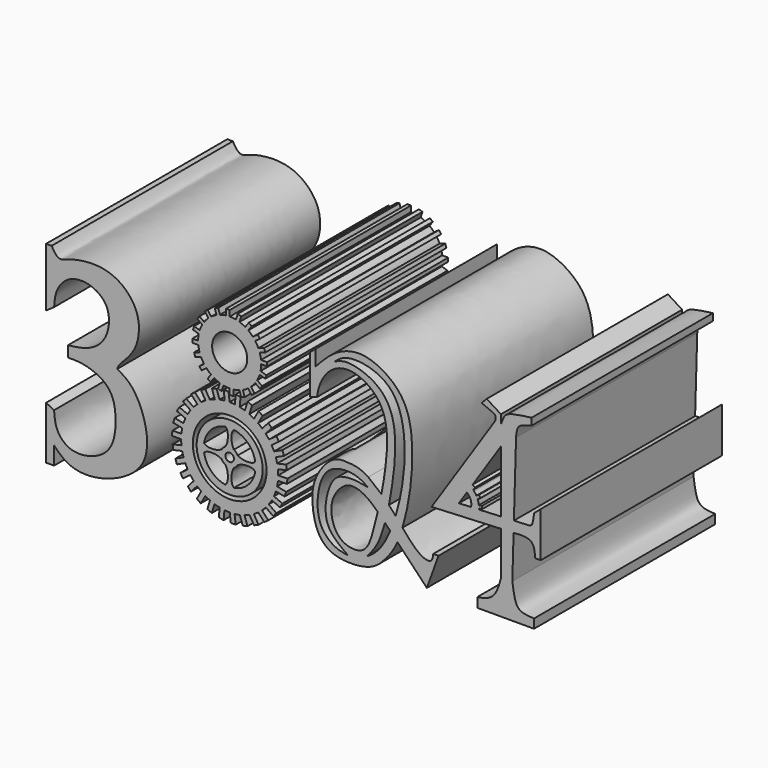
from build123d import *

# Parameters (mm, degrees)
F1_DEPTH = 25.4
F0_R     = 1.9676084545
F0_R_2   = 4.1353313865
F0_R_3   = 3.7014944741
F0_R_4   = 0.4711528495


with BuildPart() as f1:
    # F0 (on Front) → F1 (new body)
    with BuildSketch(Plane.XZ):
        with BuildLine():
            Line((-26.0463822633, -4.2281472124), (-26.9399750978, -3.781349631))
            Line((-26.9399750978, -3.781349631), (-26.9399750978, -9.7014131024))
            Line((-26.9399750978, -9.7014131024), (-26.0463822633, -9.7014131024))
            Line((-26.0463822633, -9.7014131024), (-26.0463822633, -7.6908254996))
            add(Edge.make_bspline(
                [(-26.0463822633, -7.6908254996), (-25.5832112399, -8.1670695829), (-24.5348039921, -9.2450682559), (-21.1768807028, -9.7699938511), (-15.5930362962, -7.2666656298), (-15.4178349045, -2.5163744911), (-17.1134611451, 1.0983060868), (-18.415577289, 1.8388840886), (-18.9613867551, 2.1493129898)],
                knots=[0, 0, 0, 0, 0.129274057, 0.2926173087, 0.50613754, 0.6937062734, 0.8716105194, 1, 1, 1, 1], degree=3))
            add(Edge.make_bspline(
                [(-18.9613867551, 2.1493129898), (-18.9005136877, 2.315911763), (-18.7169213448, 2.8183713956), (-16.6025126501, 4.5351279748), (-16.1925772333, 8.7200429779), (-19.1822179655, 11.5499333245), (-22.3387316619, 11.7305561988), (-24.41055806, 11.26250848), (-25.559395717, 10.6703060682), (-26.056975445, 11.4817221186), (-26.3196341693, 11.9100464508)],
                knots=[0, 0, 0, 0, 0.0677831185, 0.2044329627, 0.3733647654, 0.5392909189, 0.6902206867, 0.8157546293, 0.9027419099, 1, 1, 1, 1], degree=3))
            Line((-26.3196341693, 11.9100464508), (-26.9399750978, 11.9100464508))
            Line((-26.9399750978, 11.9100464508), (-26.9399750978, 5.3211003542))
            Line((-26.9399750978, 5.3211003542), (-26.0422043502, 5.9453165159))
            add(Edge.make_bspline(
                [(-26.0422043502, 5.9453165159), (-26.0009159793, 6.5093417381), (-25.9150413445, 7.6824434828), (-24.6120501776, 9.4535448655), (-22.1715623233, 9.7630392129), (-19.6107393646, 8.1518881576), (-19.9551089552, 4.5626923484), (-22.1437336262, 2.9722513752), (-23.7131036319, 2.7876993587), (-24.4825910777, 2.6972105261)],
                knots=[0, 0, 0, 0, 0.1221770543, 0.2541129544, 0.3944346974, 0.5457596611, 0.710117129, 0.8578657492, 1, 1, 1, 1], degree=3))
            Line((-24.4825910777, 2.6972105261), (-24.4825910777, 1.468517934))
            add(Edge.make_bspline(
                [(-26.0463822633, -4.2281472124), (-25.9967725583, -4.8661935435), (-25.8925157061, -6.2070743666), (-23.9620153869, -8.1304354588), (-19.5761648799, -6.930142804), (-18.9392916703, -3.0716265738), (-19.513902686, 0.3100528568), (-22.6669036758, 1.5162037435), (-23.9313084782, 1.4829963938), (-24.4825910777, 1.468517934)],
                knots=[0, 0, 0, 0, 0.1192071231, 0.2505187124, 0.418191993, 0.5811975133, 0.7349402199, 0.8844334945, 1, 1, 1, 1], degree=3))
        make_face()
    extrude(amount=F1_DEPTH)


with BuildPart() as f1b:
    # F0 (on Front) → F1, piece 2 (new body)
    with BuildSketch(Plane.XZ):
        with BuildLine():
            Line((-9.1431848754, 11.0277357752), (-8.7476742344, 10.4833620795))
            ThreePointArc((-8.7476742344, 10.4833620795), (-8.9926500243, 10.2350100375), (-9.2119951729, 9.9637544749))
            Line((-9.2119951729, 9.9637544749), (-9.7375776543, 10.3456124996))
            Line((-9.7375776543, 10.3456124996), (-9.9805512287, 10.0111880646))
            Line((-9.9805512287, 10.0111880646), (-9.436177533, 9.6156774235))
            ThreePointArc((-9.436177533, 9.6156774235), (-9.5924183528, 9.3037789133), (-9.717205407, 8.9780181644))
            Line((-9.717205407, 8.9780181644), (-10.3350646698, 9.1787728084))
            Line((-10.3350646698, 9.1787728084), (-10.4628034373, 8.7856333066))
            Line((-10.4628034373, 8.7856333066), (-9.8228537772, 8.5777010574))
            ThreePointArc((-9.8228537772, 8.5777010574), (-9.8750656868, 8.2327868784), (-9.8930796203, 7.8844086749))
            Line((-9.8930796203, 7.8844086749), (-10.5427352951, 7.8844086749))
            Line((-10.5427352951, 7.8844086749), (-10.5427352951, 7.4710373399))
            Line((-10.5427352951, 7.4710373399), (-9.8698524021, 7.4710373399))
            ThreePointArc((-9.8698524021, 7.4710373399), (-9.812924536, 7.126870095), (-9.7224020195, 6.7899761229))
            Line((-9.7224020195, 6.7899761229), (-10.3402612823, 6.5892214788))
            Line((-10.3402612823, 6.5892214788), (-10.2125225148, 6.196081977))
            Line((-10.2125225148, 6.196081977), (-9.5725728547, 6.4040142262))
            ThreePointArc((-9.5725728547, 6.4040142262), (-9.4120777091, 6.0942834033), (-9.2218797172, 5.8018511918))
            Line((-9.2218797172, 5.8018511918), (-9.7474621987, 5.4199931671))
            Line((-9.7474621987, 5.4199931671), (-9.5044886242, 5.0855687321))
            Line((-9.5044886242, 5.0855687321), (-8.9601149285, 5.4810793731))
            ThreePointArc((-8.9601149285, 5.4810793731), (-8.7117628865, 5.2361035832), (-8.4405073239, 5.0167584346))
            Line((-8.4405073239, 5.0167584346), (-8.8223653486, 4.4911759532))
            Line((-8.8223653486, 4.4911759532), (-8.4879409136, 4.2482023788))
            Line((-8.4879409136, 4.2482023788), (-8.0924302726, 4.7925760745))
            ThreePointArc((-8.0924302726, 4.7925760745), (-7.7805317624, 4.6363352547), (-7.4547710134, 4.5115482005))
            Line((-7.4547710134, 4.5115482005), (-7.6555256574, 3.8936889377))
            Line((-7.6555256574, 3.8936889377), (-7.2623861556, 3.7659501702))
            Line((-7.2623861556, 3.7659501702), (-7.0544539065, 4.4058998303))
            ThreePointArc((-7.0544539065, 4.4058998303), (-6.7095397274, 4.3536879207), (-6.3611615239, 4.3356739872))
            Line((-6.3611615239, 4.3356739872), (-6.3611615239, 3.6860183124))
            Line((-6.3611615239, 3.6860183124), (-5.9477901889, 3.6860183124))
            Line((-5.9477901889, 3.6860183124), (-5.9477901889, 4.3589012054))
            ThreePointArc((-5.9477901889, 4.3589012054), (-5.603622944, 4.4158290715), (-5.2667289719, 4.506351588))
            Line((-5.2667289719, 4.506351588), (-5.0659743279, 3.8884923252))
            Line((-5.0659743279, 3.8884923252), (-4.6728348261, 4.0162310927))
            Line((-4.6728348261, 4.0162310927), (-4.8807670752, 4.6561807528))
            ThreePointArc((-4.8807670752, 4.6561807528), (-4.5710362523, 4.8166758984), (-4.2786040408, 5.0068738902))
            Line((-4.2786040408, 5.0068738902), (-3.8967460161, 4.4812914088))
            Line((-3.8967460161, 4.4812914088), (-3.5623215811, 4.7242649833))
            Line((-3.5623215811, 4.7242649833), (-3.9578322221, 5.268638679))
            ThreePointArc((-3.9578322221, 5.268638679), (-3.7128564322, 5.516990721), (-3.4935112837, 5.7882462836))
            Line((-3.4935112837, 5.7882462836), (-2.9679288023, 5.4063882589))
            Line((-2.9679288023, 5.4063882589), (-2.7249552278, 5.7408126939))
            Line((-2.7249552278, 5.7408126939), (-3.2693289235, 6.1363233349))
            ThreePointArc((-3.2693289235, 6.1363233349), (-3.1130881037, 6.4482218451), (-2.9883010496, 6.7739825941))
            Line((-2.9883010496, 6.7739825941), (-2.3704417867, 6.5732279501))
            Line((-2.3704417867, 6.5732279501), (-2.2427030192, 6.9663674519))
            Line((-2.2427030192, 6.9663674519), (-2.8826526793, 7.174299701))
            ThreePointArc((-2.8826526793, 7.174299701), (-2.8304407697, 7.5192138801), (-2.8124268362, 7.8675920836))
            Line((-2.8124268362, 7.8675920836), (-2.1627711614, 7.8675920836))
            Line((-2.1627711614, 7.8675920836), (-2.1627711614, 8.2809634186))
            Line((-2.1627711614, 8.2809634186), (-2.8356540545, 8.2809634186))
            ThreePointArc((-2.8356540545, 8.2809634186), (-2.8925819205, 8.6251306635), (-2.983104437, 8.9620246356))
            Line((-2.983104437, 8.9620246356), (-2.3652451742, 9.1627792796))
            Line((-2.3652451742, 9.1627792796), (-2.4929839417, 9.5559187814))
            Line((-2.4929839417, 9.5559187814), (-3.1329336018, 9.3479865323))
            ThreePointArc((-3.1329336018, 9.3479865323), (-3.2934287474, 9.6577173552), (-3.4836267393, 9.9501495667))
            Line((-3.4836267393, 9.9501495667), (-2.9580442579, 10.3320075914))
            Line((-2.9580442579, 10.3320075914), (-3.2010178323, 10.6664320264))
            Line((-3.2010178323, 10.6664320264), (-3.745391528, 10.2709213854))
            ThreePointArc((-3.745391528, 10.2709213854), (-3.99374357, 10.5158971753), (-4.2649991326, 10.7352423238))
            Line((-4.2649991326, 10.7352423238), (-3.8831411079, 11.2608248052))
            Line((-3.8831411079, 11.2608248052), (-4.2175655429, 11.5037983797))
            Line((-4.2175655429, 11.5037983797), (-4.613076184, 10.959424684))
            ThreePointArc((-4.613076184, 10.959424684), (-4.9249746942, 11.1156655038), (-5.2507354431, 11.2404525579))
            Line((-5.2507354431, 11.2404525579), (-5.0499807991, 11.8583118208))
            Line((-5.0499807991, 11.8583118208), (-5.4431203009, 11.9860505883))
            Line((-5.4431203009, 11.9860505883), (-5.6510525501, 11.3461009282))
            ThreePointArc((-5.6510525501, 11.3461009282), (-5.9959667291, 11.3983128378), (-6.3443449326, 11.4163267713))
            Line((-6.3443449326, 11.4163267713), (-6.3443449326, 11.393099553))
            Line((-6.3443449326, 11.393099553), (-6.7577162676, 11.393099553))
            ThreePointArc((-6.7577162676, 11.393099553), (-7.1018835125, 11.336171687), (-7.4387774846, 11.2456491705))
            Line((-7.4387774846, 11.2456491705), (-7.6395321286, 11.8635084333))
            Line((-7.6395321286, 11.8635084333), (-8.0326716305, 11.7357696658))
            Line((-8.0326716305, 11.7357696658), (-7.8247393813, 11.0958200057))
            ThreePointArc((-7.8247393813, 11.0958200057), (-8.1344702042, 10.9353248601), (-8.4269024157, 10.7451268682))
            Line((-8.4269024157, 10.7451268682), (-8.8087604404, 11.2707093496))
            Line((-8.8087604404, 11.2707093496), (-9.1431848754, 11.0277357752))
        make_face()
        with Locations((-6.3527532283, 7.8760003792)):
            Circle(F0_R, mode=Mode.SUBTRACT)
        Polygon((-6.7577162676, 12.0659824461), (-6.7577162676, 11.393099553), (-6.3443449326, 11.393099553), (-6.3443449326, 11.4163267713), (-6.3443449326, 12.0659824461), align=None)
    extrude(amount=F1_DEPTH)


with BuildPart() as f1c:
    # F0 (on Front) → F1, piece 3 (new body)
    with BuildSketch(Plane.XZ):
        with BuildLine():
            Line((-8.3493689741, 3.6920308456), (-8.0175920904, 2.7096574241))
            ThreePointArc((-8.0175920904, 2.7096574241), (-8.2983395388, 2.6108656256), (-8.5732644732, 2.4968690045))
            Line((-8.5732644732, 2.4968690045), (-9.087648101, 3.3645220331))
            Line((-9.087648101, 3.3645220331), (-9.5868565309, 3.1422601201))
            Line((-9.5868565309, 3.1422601201), (-9.0580828491, 2.2503342077))
            ThreePointArc((-9.0580828491, 2.2503342077), (-9.3121553223, 2.0953305703), (-9.5573712571, 1.926664941))
            Line((-9.5573712571, 1.926664941), (-10.2409095766, 2.6684112994))
            Line((-10.2409095766, 2.6684112994), (-10.6829982545, 2.3472150737))
            Line((-10.6829982545, 2.3472150737), (-9.9803377218, 1.5847181127))
            ThreePointArc((-9.9803377218, 1.5847181127), (-10.1966310335, 1.3802770392), (-10.4014208556, 1.1643138989))
            Line((-10.4014208556, 1.1643138989), (-11.2242399624, 1.747735712))
            Line((-11.2242399624, 1.747735712), (-11.5898874916, 1.34164299))
            Line((-11.5898874916, 1.34164299), (-10.744049745, 0.7418997564))
            ThreePointArc((-10.744049745, 0.7418997564), (-10.9131108396, 0.4969563028), (-11.0685242511, 0.243134277))
            Line((-11.0685242511, 0.243134277), (-11.9946630019, 0.642733212))
            Line((-11.9946630019, 0.642733212), (-12.2678888309, 0.1694921942))
            Line((-12.2678888309, 0.1694921942), (-11.3158410386, -0.2412856547))
            ThreePointArc((-11.3158410386, -0.2412856547), (-11.4302811351, -0.5160262842), (-11.5295258242, -0.7966139548))
            Line((-11.5295258242, -0.7966139548), (-12.5185075114, -0.598302289))
            Line((-12.5185075114, -0.598302289), (-12.6873703603, -1.1180086992))
            Line((-12.6873703603, -1.1180086992), (-11.6707215794, -1.3218682002))
            ThreePointArc((-11.6707215794, -1.3218682002), (-11.7255390964, -1.6143985218), (-11.7642775939, -1.9094888097))
            Line((-11.7642775939, -1.9094888097), (-12.7728789721, -1.9211315843))
            Line((-12.7728789721, -1.9211315843), (-12.8299987242, -2.464589723))
            Line((-12.8299987242, -2.464589723), (-11.7931813849, -2.4526212379))
            ThreePointArc((-11.7931813849, -2.4526212379), (-11.7859805338, -2.7501562727), (-11.7625197814, -3.0468523164))
            Line((-11.7625197814, -3.0468523164), (-12.7466601307, -3.2679406863))
            Line((-12.7466601307, -3.2679406863), (-12.6895403787, -3.811398825))
            Line((-12.6895403787, -3.811398825), (-11.6778683738, -3.5841254339))
            ThreePointArc((-11.6778683738, -3.5841254339), (-11.6089638664, -3.8736614732), (-11.5243292117, -4.1589962317))
            Line((-11.5243292117, -4.1589962317), (-12.4409968763, -4.5798675744))
            Line((-12.4409968763, -4.5798675744), (-12.2721340274, -5.0995739846))
            Line((-12.2721340274, -5.0995739846), (-11.3298222781, -4.6669286253))
            ThreePointArc((-11.3298222781, -4.6669286253), (-11.202225572, -4.9358115549), (-11.0601159554, -5.1973145302))
            Line((-11.0601159554, -5.1973145302), (-11.8692481598, -5.7995747482))
            Line((-11.8692481598, -5.7995747482), (-11.5960223308, -6.272815766))
            Line((-11.5960223308, -6.272815766), (-10.7642543823, -5.6537071168))
            ThreePointArc((-10.7642543823, -5.6537071168), (-10.5835420658, -5.8901854623), (-10.3901683596, -6.1164277195))
            Line((-10.3901683596, -6.1164277195), (-11.0564021437, -6.8737551516))
            Line((-11.0564021437, -6.8737551516), (-10.6907546145, -7.2798478736))
            Line((-10.6907546145, -7.2798478736), (-10.0058827173, -6.5013339532))
            ThreePointArc((-10.0058827173, -6.5013339532), (-9.7799527859, -6.6950724763), (-9.5437663489, -6.8761661431))
            Line((-9.5437663489, -6.8761661431), (-10.0379840994, -7.7554619463))
            Line((-10.0379840994, -7.7554619463), (-9.5958954215, -8.076658172))
            Line((-9.5958954215, -8.076658172), (-9.087851764, -7.1727637745))
            ThreePointArc((-9.087851764, -7.1727637745), (-8.8265784398, -7.3152951719), (-8.5579017526, -7.4433255862))
            Line((-8.5579017526, -7.4433255862), (-8.8585037824, -8.4061603146))
            Line((-8.8585037824, -8.4061603146), (-8.3592953524, -8.6284222275))
            Line((-8.3592953524, -8.6284222275), (-8.0502838802, -7.6386518755))
            ThreePointArc((-8.0502838802, -7.6386518755), (-7.7650860612, -7.7237468413), (-7.4756615843, -7.7931184595))
            Line((-7.4756615843, -7.7931184595), (-7.5695101422, -8.7974116153))
            Line((-7.5695101422, -8.7974116153), (-7.034999764, -8.9110253034))
            Line((-7.034999764, -8.9110253034), (-6.9385257613, -7.8786367106))
            ThreePointArc((-6.9385257613, -7.8786367106), (-6.6418679606, -7.9025761865), (-6.3443449326, -7.9102571361))
            Line((-6.3443449326, -7.9102571361), (-6.2273383862, -8.9121162891))
            Line((-6.2273383862, -8.9121162891), (-5.6808867282, -8.9121162891))
            Line((-5.6808867282, -8.9121162891), (-5.8011665719, -7.882229791))
            ThreePointArc((-5.8011665719, -7.882229791), (-5.506014159, -7.843967507), (-5.2133957637, -7.7896220936))
            Line((-5.2133957637, -7.7896220936), (-4.8906478606, -8.7452611915))
            Line((-4.8906478606, -8.7452611915), (-4.3561374824, -8.6316475034))
            Line((-4.3561374824, -8.6316475034), (-4.6879143661, -7.6492740819))
            ThreePointArc((-4.6879143661, -7.6492740819), (-4.4071669178, -7.5504822834), (-4.1322419833, -7.4364856623))
            Line((-4.1322419833, -7.4364856623), (-3.6178583556, -8.3041386909))
            Line((-3.6178583556, -8.3041386909), (-3.1186499256, -8.0818767779))
            Line((-3.1186499256, -8.0818767779), (-3.6474236074, -7.1899508655))
            ThreePointArc((-3.6474236074, -7.1899508655), (-3.3933511342, -7.0349472281), (-3.1481351994, -6.8662815988))
            Line((-3.1481351994, -6.8662815988), (-2.4645968799, -7.6080279572))
            Line((-2.4645968799, -7.6080279572), (-2.022508202, -7.2868317315))
            Line((-2.022508202, -7.2868317315), (-2.7251687347, -6.5243347705))
            ThreePointArc((-2.7251687347, -6.5243347705), (-2.508875423, -6.319893697), (-2.3040856009, -6.1039305567))
            Line((-2.3040856009, -6.1039305567), (-1.4812664942, -6.6873523698))
            Line((-1.4812664942, -6.6873523698), (-1.1156189649, -6.2812596477))
            Line((-1.1156189649, -6.2812596477), (-1.9614567115, -5.6815164142))
            ThreePointArc((-1.9614567115, -5.6815164142), (-1.7923956169, -5.4365729606), (-1.6369822054, -5.1827509348))
            Line((-1.6369822054, -5.1827509348), (-0.7108434547, -5.5823498698))
            Line((-0.7108434547, -5.5823498698), (-0.4376176257, -5.109108852))
            Line((-0.4376176257, -5.109108852), (-1.3896654179, -4.6983310031))
            ThreePointArc((-1.3896654179, -4.6983310031), (-1.2752253214, -4.4235903736), (-1.1759806323, -4.143002703))
            Line((-1.1759806323, -4.143002703), (-0.1869989452, -4.3413143688))
            Line((-0.1869989452, -4.3413143688), (-0.0181360962, -3.8216079586))
            Line((-0.0181360962, -3.8216079586), (-1.0347848771, -3.6177484575))
            ThreePointArc((-1.0347848771, -3.6177484575), (-0.9799673601, -3.325218136), (-0.9412288626, -3.030127848))
            Line((-0.9412288626, -3.030127848), (0.0673725156, -3.0184850734))
            Line((0.0673725156, -3.0184850734), (0.1244922677, -2.4750269348))
            Line((0.1244922677, -2.4750269348), (-0.9123250717, -2.4869954199))
            ThreePointArc((-0.9123250717, -2.4869954199), (-0.9195259227, -2.1894603851), (-0.9429866751, -1.8927643414))
            Line((-0.9429866751, -1.8927643414), (0.0411536742, -1.6716759715))
            Line((0.0411536742, -1.6716759715), (-0.0159660779, -1.1282178328))
            Line((-0.0159660779, -1.1282178328), (-1.0276380828, -1.3554912239))
            ThreePointArc((-1.0276380828, -1.3554912239), (-1.0965425901, -1.0659551846), (-1.1811772449, -0.7806204261))
            Line((-1.1811772449, -0.7806204261), (-0.2645095802, -0.3597490834))
            Line((-0.2645095802, -0.3597490834), (-0.4333724292, 0.1599573268))
            Line((-0.4333724292, 0.1599573268), (-1.3756841785, -0.2726880325))
            ThreePointArc((-1.3756841785, -0.2726880325), (-1.5032808845, -0.0038051029), (-1.6453905011, 0.2576978724))
            Line((-1.6453905011, 0.2576978724), (-0.8362582967, 0.8599580905))
            Line((-0.8362582967, 0.8599580905), (-1.1094841257, 1.3331991082))
            Line((-1.1094841257, 1.3331991082), (-1.9412520743, 0.714090459))
            ThreePointArc((-1.9412520743, 0.714090459), (-2.1219643907, 0.9505688045), (-2.3153380969, 1.1768110617))
            Line((-2.3153380969, 1.1768110617), (-1.6491043128, 1.9341384938))
            Line((-1.6491043128, 1.9341384938), (-2.0147518421, 2.3402312158))
            Line((-2.0147518421, 2.3402312158), (-2.6996237392, 1.5617172954))
            ThreePointArc((-2.6996237392, 1.5617172954), (-2.9255536706, 1.7554558185), (-3.1617401076, 1.9365494853))
            Line((-3.1617401076, 1.9365494853), (-2.6675223571, 2.8158452885))
            Line((-2.6675223571, 2.8158452885), (-3.109611035, 3.1370415142))
            Line((-3.109611035, 3.1370415142), (-3.6176546925, 2.2331471167))
            ThreePointArc((-3.6176546925, 2.2331471167), (-3.8789280167, 2.3756785141), (-4.1476047039, 2.5037089284))
            Line((-4.1476047039, 2.5037089284), (-3.8470026741, 3.4665436568))
            Line((-3.8470026741, 3.4665436568), (-4.3462111041, 3.6888055697))
            Line((-4.3462111041, 3.6888055697), (-4.6552225763, 2.6990352177))
            ThreePointArc((-4.6552225763, 2.6990352177), (-4.9404203953, 2.7841301835), (-5.2298448722, 2.8535018017))
            Line((-5.2298448722, 2.8535018017), (-5.1359963143, 3.8577949575))
            Line((-5.1359963143, 3.8577949575), (-5.6705066925, 3.9714086456))
            Line((-5.6705066925, 3.9714086456), (-5.7669806952, 2.9390200528))
            ThreePointArc((-5.7669806952, 2.9390200528), (-6.0636384959, 2.9629595287), (-6.3611615239, 2.9706404783))
            Line((-6.3611615239, 2.9706404783), (-6.4781680703, 3.9724996313))
            Line((-6.4781680703, 3.9724996313), (-7.0246197283, 3.9724996313))
            Line((-7.0246197283, 3.9724996313), (-6.9043398847, 2.9426131332))
            ThreePointArc((-6.9043398847, 2.9426131332), (-7.1994922975, 2.9043508492), (-7.4921106928, 2.8500054358))
            Line((-7.4921106928, 2.8500054358), (-7.8148585959, 3.8056445337))
            Line((-7.8148585959, 3.8056445337), (-8.3493689741, 3.6920308456))
        make_face()
        with Locations((-6.3527532283, -2.4698083289)):
            Circle(F0_R_2, mode=Mode.SUBTRACT)
    extrude(amount=F1_DEPTH)


with BuildPart() as f1d:
    # F0 (on Front) → F1, piece 4 (new body)
    with BuildSketch(Plane.XZ):
        with Locations((-6.3527532283, -2.4698083289)):
            Circle(F0_R_3)
        with BuildLine():
            add(Edge.make_bspline(
                [(-7.2560629998, -2.9409611784), (-7.4238569383, -2.8554461757), (-7.8043314459, -2.6615400144), (-8.8419767294, -2.6416756573), (-9.1140801532, -2.8547030748), (-9.2242590475, -2.9409611784)],
                knots=[0, 0, 0, 0, 0.3194921696, 0.7244518306, 1, 1, 1, 1], degree=3))
            ThreePointArc((-7.2560629998, -2.9409611784), (-7.0731536554, -3.1902087561), (-6.8239060777, -3.3731181005))
            add(Edge.make_bspline(
                [(-6.8239060777, -3.3731181005), (-6.7383910751, -3.5409120389), (-6.5444849137, -3.9213865465), (-6.5246205566, -4.9590318301), (-6.7376479741, -5.2311352538), (-6.8239060777, -5.3413141481)],
                knots=[0, 0, 0, 0, 0.3194921696, 0.7244518306, 1, 1, 1, 1], degree=3))
            ThreePointArc((-6.8239060777, -5.3413141481), (-8.4103647899, -4.5274198906), (-9.2242590475, -2.9409611784))
        make_face(mode=Mode.SUBTRACT)
        with Locations((-6.3527532283, -2.4698083289)):
            Circle(F0_R_4, mode=Mode.SUBTRACT)
        with BuildLine():
            add(Edge.make_bspline(
                [(-5.8816003788, -3.3731181005), (-5.9671153814, -3.5409120389), (-6.1610215428, -3.9213865465), (-6.1808858999, -4.9590318301), (-5.9678584824, -5.2311352538), (-5.8816003788, -5.3413141481)],
                knots=[0, 0, 0, 0, 0.3194921696, 0.7244518306, 1, 1, 1, 1], degree=3))
            ThreePointArc((-5.8816003788, -3.3731181005), (-5.6323528011, -3.1902087561), (-5.4494434567, -2.9409611784))
            add(Edge.make_bspline(
                [(-5.4494434567, -2.9409611784), (-5.2816495182, -2.8554461757), (-4.9011750106, -2.6615400144), (-3.8635297271, -2.6416756573), (-3.5914263033, -2.8547030748), (-3.481247409, -2.9409611784)],
                knots=[0, 0, 0, 0, 0.3194921696, 0.7244518306, 1, 1, 1, 1], degree=3))
            ThreePointArc((-3.481247409, -2.9409611784), (-4.2951416666, -4.5274198906), (-5.8816003788, -5.3413141481))
        make_face(mode=Mode.SUBTRACT)
        with BuildLine():
            ThreePointArc((-9.2242590475, -1.9986554794), (-8.4103647899, -0.4121967672), (-6.8239060777, 0.4016974903))
            add(Edge.make_bspline(
                [(-6.8239060777, -1.5664985573), (-6.7383910751, -1.3987046188), (-6.5444849137, -1.0182301113), (-6.5246205566, 0.0194151723), (-6.7376479741, 0.2915185961), (-6.8239060777, 0.4016974903)],
                knots=[0, 0, 0, 0, 0.3194921696, 0.7244518306, 1, 1, 1, 1], degree=3))
            ThreePointArc((-6.8239060777, -1.5664985573), (-7.0731536554, -1.7494079017), (-7.2560629998, -1.9986554794))
            add(Edge.make_bspline(
                [(-7.2560629998, -1.9986554794), (-7.4238569383, -2.0841704821), (-7.8043314459, -2.2780766434), (-8.8419767294, -2.2979410005), (-9.1140801532, -2.084913583), (-9.2242590475, -1.9986554794)],
                knots=[0, 0, 0, 0, 0.3194921696, 0.7244518306, 1, 1, 1, 1], degree=3))
        make_face(mode=Mode.SUBTRACT)
        with BuildLine():
            ThreePointArc((-5.4494434567, -1.9986554794), (-5.6323528011, -1.7494079017), (-5.8816003788, -1.5664985573))
            add(Edge.make_bspline(
                [(-5.8816003788, -1.5664985573), (-5.9671153814, -1.3987046188), (-6.1610215428, -1.0182301113), (-6.1808858999, 0.0194151723), (-5.9678584824, 0.2915185961), (-5.8816003788, 0.4016974903)],
                knots=[0, 0, 0, 0, 0.3194921696, 0.7244518306, 1, 1, 1, 1], degree=3))
            ThreePointArc((-5.8816003788, 0.4016974903), (-4.2951416666, -0.4121967672), (-3.481247409, -1.9986554794))
            add(Edge.make_bspline(
                [(-5.4494434567, -1.9986554794), (-5.2816495182, -2.0841704821), (-4.9011750106, -2.2780766434), (-3.8635297271, -2.2979410005), (-3.5914263033, -2.084913583), (-3.481247409, -1.9986554794)],
                knots=[0, 0, 0, 0, 0.3194921696, 0.7244518306, 1, 1, 1, 1], degree=3))
        make_face(mode=Mode.SUBTRACT)
    extrude(amount=F1_DEPTH)


with BuildPart() as f1e:
    # F0 (on Front) → F1, piece 5 (new body)
    with BuildSketch(Plane.XZ):
        with BuildLine():
            Line((2.6719989255, 10.845345445), (2.6719989255, 6.3930512406))
            Line((2.6719989255, 6.3930512406), (3.435845949, 6.6561674627))
            add(Edge.make_bspline(
                [(3.435845949, 6.6561674627), (3.4947846069, 7.0290440395), (3.631181329, 7.891960582), (4.6469745705, 9.8721275201), (7.2502428175, 10.9905601524), (11.4292677124, 8.5643622597), (11.4047338514, 3.7879569996), (10.8541188192, 0.4220713966), (10.662418889, -0.5672860666)],
                knots=[0, 0, 0, 0, 0.0554862745, 0.1284071651, 0.2079981655, 0.3080730139, 0.4305049606, 0.4841391387, 0.4841391387, 0.4841391387, 0.4841391387], degree=3))
            add(Edge.make_bspline(
                [(11.5063009471, -1.3741382079), (11.2197324238, -1.0774084626), (10.9391479112, -0.8121944395), (10.6624189097, -0.5672860636)],
                knots=[0.7225338292, 0.7225338292, 0.7225338292, 0.7225338292, 0.8212279518, 0.8212279518, 0.8212279518, 0.8212279518], degree=3))
            add(Edge.make_bspline(
                [(5.3971023299, 10.8085060492), (5.7772404462, 10.972500295), (6.6584668398, 11.3526675333), (8.9599957978, 10.8384738524), (11.1535014908, 9.4534977213), (12.5082732699, 6.2739507893), (12.0837887958, 1.7807829115), (11.5957909908, -0.9246608458), (11.5063009471, -1.3741382079)],
                knots=[0, 0, 0, 0, 0.0918839164, 0.2130029292, 0.3401946496, 0.4838683251, 0.688082351, 0.7299642077, 0.7299642077, 0.7299642077, 0.7299642077], degree=3))
            add(Edge.make_bspline(
                [(5.3971023299, 10.8085060492), (5.7620619847, 11.1079679478), (6.609363119, 11.8051385726), (9.3198931691, 11.7283905399), (12.668565724, 10.0341568395), (13.6683514535, 4.5184758873), (12.8192457315, -0.3650505129), (12.261372983, -2.2119843023)],
                knots=[0, 0, 0, 0, 0.1014740063, 0.2350549924, 0.3880747556, 0.5958223129, 0.7618945915, 0.7618945915, 0.7618945915, 0.7618945915], degree=3))
            add(Edge.make_bspline(
                [(13.0264212728, -3.1206628495), (12.7704039085, -2.8165986405), (12.5144389833, -2.5076877064), (12.261372983, -2.2119843023)],
                knots=[0.5530933365, 0.5530933365, 0.5530933365, 0.5530933365, 0.6373963086, 0.6373963086, 0.6373963086, 0.6373963086], degree=3))
            add(Edge.make_bspline(
                [(13.0264212728, -3.1206628495), (13.0837947511, -2.9258450596), (13.4575273646, -1.5863706141), (14.0352558584, 1.2503294705), (14.2882363414, 6.1221826163), (13.2278084517, 10.4171777534), (8.9691725141, 12.9168064821), (6.1016622002, 12.1680848808), (4.5226306163, 10.9638438122), (3.6928214025, 10.0698512074), (3.2855544844, 9.6310833469)],
                knots=[0.5451714575, 0.5451714575, 0.5451714575, 0.5451714575, 0.5569891983, 0.6250982674, 0.7020008511, 0.773863392, 0.847306886, 0.9050067166, 0.9533388622, 1, 1, 1, 1], degree=3))
            Line((3.2855544844, 9.6310833469), (3.2855544844, 11.3618402075))
            Line((3.2855544844, 11.3618402075), (2.6719989255, 10.845345445))
        make_face()
        with BuildLine():
            add(Edge.make_bspline(
                [(10.662418889, -0.5672860666), (10.5354882317, -1.2223712975), (10.3980492387, -1.8616839287), (10.2575550909, -2.466147512)],
                knots=[0.4841391387, 0.4841391387, 0.4841391387, 0.4841391387, 0.519652044, 0.519652044, 0.519652044, 0.519652044], degree=3))
            add(Edge.make_bspline(
                [(10.6624189097, -0.5672860636), (10.1611589652, -0.1236651991), (9.6725492558, 0.253331238), (9.1839395463, 0.630327675)],
                knots=[0.8212279518, 0.8212279518, 0.8212279518, 0.8212279518, 1, 1, 1, 1], degree=3))
            add(Edge.make_bspline(
                [(9.1839395463, 0.630327675), (8.3293113858, 1.2043820461), (7.0371029965, 1.3526036912), (5.0848852762, 1.4045628888), (2.9521080111, -1.3902184626), (2.8538912632, -4.0498435296), (3.2760692481, -6.416794074), (4.8429420361, -8.6433503566), (9.3575740444, -8.6163306128), (11.0399209282, -6.984464507), (11.9734456221, -5.7662631109), (12.3803034392, -4.9061127741), (12.4598010347, -4.7229557439)],
                knots=[0, 0, 0, 0, 0.0530742276, 0.0986896089, 0.1608436336, 0.217710048, 0.2707461549, 0.3252123246, 0.3955657221, 0.4477864087, 0.4977663247, 0.5106388975, 0.5106388975, 0.5106388975, 0.5106388975], degree=3))
            add(Edge.make_bspline(
                [(12.4598010347, -4.7229557439), (12.1935596674, -4.4485073887), (11.9253475631, -4.171569745), (11.6621594556, -3.8986119129)],
                knots=[0.448384843, 0.448384843, 0.448384843, 0.448384843, 0.5312386615, 0.5312386615, 0.5312386615, 0.5312386615], degree=3))
            add(Edge.make_bspline(
                [(11.6621594556, -3.8986119129), (11.5577343223, -4.1480369004), (10.7999785534, -5.8142653195), (9.895978436, -6.779659418), (9.0104155242, -7.2580603883)],
                knots=[0.8160688803, 0.8160688803, 0.8160688803, 0.8160688803, 0.8422565533, 1, 1, 1, 1], degree=3))
            add(Edge.make_bspline(
                [(11.0650681475, -3.2797242735), (10.837325615, -4.1199552873), (10.2295225901, -5.8875703382), (9.4570090084, -6.7560110248), (9.0104155242, -7.2580603883)],
                knots=[0.7921233606, 0.7921233606, 0.7921233606, 0.7921233606, 0.8798256046, 1, 1, 1, 1], degree=3))
            add(Edge.make_bspline(
                [(11.0650681475, -3.2797242735), (10.7861687813, -2.99207196), (10.515826503, -2.7171147888), (10.2575550909, -2.466147512)],
                knots=[0.594962196, 0.594962196, 0.594962196, 0.594962196, 0.6859914774, 0.6859914774, 0.6859914774, 0.6859914774], degree=3))
        make_face()
        with BuildLine():
            add(Edge.make_bspline(
                [(10.2575550909, -2.466147512), (9.8682447349, -2.087847184), (9.0400940624, -1.3468679748), (8.4186032489, -1.093940724), (8.0686900765, -0.9515370475)],
                knots=[0.6859914774, 0.6859914774, 0.6859914774, 0.6859914774, 0.8232062069, 1, 1, 1, 1], degree=3))
            add(Edge.make_bspline(
                [(10.2575550909, -2.466147512), (10.0773075767, -3.2416464209), (9.5669102142, -5.2199681104), (8.8961666731, -7.1539738384), (6.3422217324, -7.0283640709), (5.0450398017, -5.2742443341), (4.8964332472, -2.6360270309), (6.7214277914, -0.6676655418), (7.670389297, -0.8676140852), (8.0686900765, -0.9515370475)],
                knots=[0.519652044, 0.519652044, 0.519652044, 0.519652044, 0.5652134642, 0.6451642659, 0.7158366661, 0.7872018805, 0.8671122417, 0.9442239781, 1, 1, 1, 1], degree=3))
        make_face(mode=Mode.SUBTRACT)
        with BuildLine():
            add(Edge.make_bspline(
                [(9.1839395463, -0.3927653015), (8.7034378735, -0.0827222792), (7.644212587, 0.6007413332), (4.6295094071, 0.397337352), (3.3778114221, -2.438787929), (3.4790722413, -6.0078719774), (5.464417191, -7.6423112234), (6.4526749104, -7.7662268961), (6.8825753406, -7.8201312572)],
                knots=[0, 0, 0, 0, 0.1459435349, 0.3217201757, 0.5048827787, 0.7071792002, 0.8726204862, 1, 1, 1, 1], degree=3))
            add(Edge.make_bspline(
                [(9.1839395463, -0.3927653015), (8.601031245, -0.2801566836), (7.4842634033, -0.0644148886), (5.9216849775, -0.287488793), (5.2088825786, -0.9417540787), (4.4636091166, -2.4754982841), (4.158334886, -5.8528096932), (5.9696811872, -7.1608809511), (6.8825753406, -7.8201312572)],
                knots=[0, 0, 0, 0, 0.1601804553, 0.3068825422, 0.4193280853, 0.5742172296, 0.7854112152, 1, 1, 1, 1], degree=3))
        make_face(mode=Mode.SUBTRACT)
        with BuildLine():
            add(Edge.make_bspline(
                [(11.5063009471, -1.3741382079), (11.2197324238, -1.0774084626), (10.9391479112, -0.8121944395), (10.6624189097, -0.5672860636)],
                knots=[0.7225338292, 0.7225338292, 0.7225338292, 0.7225338292, 0.8212279518, 0.8212279518, 0.8212279518, 0.8212279518], degree=3))
            add(Edge.make_bspline(
                [(10.662418889, -0.5672860666), (10.5354882317, -1.2223712975), (10.3980492387, -1.8616839287), (10.2575550909, -2.466147512)],
                knots=[0.4841391387, 0.4841391387, 0.4841391387, 0.4841391387, 0.519652044, 0.519652044, 0.519652044, 0.519652044], degree=3))
            add(Edge.make_bspline(
                [(11.0650681475, -3.2797242735), (10.7861687813, -2.99207196), (10.515826503, -2.7171147888), (10.2575550909, -2.466147512)],
                knots=[0.594962196, 0.594962196, 0.594962196, 0.594962196, 0.6859914774, 0.6859914774, 0.6859914774, 0.6859914774], degree=3))
            add(Edge.make_bspline(
                [(11.5063009471, -1.3741382079), (11.3734838813, -2.0412321318), (11.2264811545, -2.6842087458), (11.0650681475, -3.2797242735)],
                knots=[0.7299642077, 0.7299642077, 0.7299642077, 0.7299642077, 0.7921233606, 0.7921233606, 0.7921233606, 0.7921233606], degree=3))
        make_face()
        with BuildLine():
            add(Edge.make_bspline(
                [(12.261372983, -2.2119843023), (12.0911548955, -2.0130873037), (11.8375528818, -1.7234282501), (11.5888601796, -1.4596248474), (11.5063009471, -1.3741382079)],
                knots=[0.6373963086, 0.6373963086, 0.6373963086, 0.6373963086, 0.6941004517, 0.7225338292, 0.7225338292, 0.7225338292, 0.7225338292], degree=3))
            add(Edge.make_bspline(
                [(11.5063009471, -1.3741382079), (11.3734838813, -2.0412321318), (11.2264811545, -2.6842087458), (11.0650681475, -3.2797242735)],
                knots=[0.7299642077, 0.7299642077, 0.7299642077, 0.7299642077, 0.7921233606, 0.7921233606, 0.7921233606, 0.7921233606], degree=3))
            add(Edge.make_bspline(
                [(11.6621594556, -3.8986119129), (11.6605063562, -3.8968974492), (11.4581105476, -3.6869826231), (11.2587125577, -3.4794459988), (11.0650681475, -3.2797242735)],
                knots=[0.5312386615, 0.5312386615, 0.5312386615, 0.5312386615, 0.5317590711, 0.594962196, 0.594962196, 0.594962196, 0.594962196], degree=3))
            add(Edge.make_bspline(
                [(12.261372983, -2.2119843023), (12.0793898147, -2.8144709152), (11.8781831296, -3.3826278725), (11.6621594556, -3.8986119129)],
                knots=[0.7618945915, 0.7618945915, 0.7618945915, 0.7618945915, 0.8160688803, 0.8160688803, 0.8160688803, 0.8160688803], degree=3))
        make_face()
        with BuildLine():
            add(Edge.make_bspline(
                [(12.4598010347, -4.7229557439), (12.6730649672, -4.2316102095), (12.8587705255, -3.6899389172), (13.0264212728, -3.1206628495)],
                knots=[0.5106388975, 0.5106388975, 0.5106388975, 0.5106388975, 0.5451714575, 0.5451714575, 0.5451714575, 0.5451714575], degree=3))
            add(Edge.make_bspline(
                [(13.0264212728, -3.1206628495), (12.7704039085, -2.8165986405), (12.5144389833, -2.5076877064), (12.261372983, -2.2119843023)],
                knots=[0.5530933365, 0.5530933365, 0.5530933365, 0.5530933365, 0.6373963086, 0.6373963086, 0.6373963086, 0.6373963086], degree=3))
            add(Edge.make_bspline(
                [(12.261372983, -2.2119843023), (12.0793898147, -2.8144709152), (11.8781831296, -3.3826278725), (11.6621594556, -3.8986119129)],
                knots=[0.7618945915, 0.7618945915, 0.7618945915, 0.7618945915, 0.8160688803, 0.8160688803, 0.8160688803, 0.8160688803], degree=3))
            add(Edge.make_bspline(
                [(12.4598010347, -4.7229557439), (12.1935596674, -4.4485073887), (11.9253475631, -4.171569745), (11.6621594556, -3.8986119129)],
                knots=[0.448384843, 0.448384843, 0.448384843, 0.448384843, 0.5312386615, 0.5312386615, 0.5312386615, 0.5312386615], degree=3))
        make_face()
        with BuildLine():
            add(Edge.make_bspline(
                [(16.4786074311, -4.5802788809), (16.4439176157, -4.8929619563), (16.3652489872, -5.6020562102), (14.9131623086, -5.3009986325), (13.6836853528, -3.9012758484), (13.0264212728, -3.1206628495)],
                knots=[0, 0, 0, 0, 0.1484563798, 0.3366653784, 0.5530933365, 0.5530933365, 0.5530933365, 0.5530933365], degree=3))
            add(Edge.make_bspline(
                [(12.4598010347, -4.7229557439), (12.6730649672, -4.2316102095), (12.8587705255, -3.6899389172), (13.0264212728, -3.1206628495)],
                knots=[0.5106388975, 0.5106388975, 0.5106388975, 0.5106388975, 0.5451714575, 0.5451714575, 0.5451714575, 0.5451714575], degree=3))
            add(Edge.make_bspline(
                [(15.7590452582, -8.1780925393), (15.3984665019, -7.7867808083), (14.6325807763, -6.9556168423), (13.222290813, -5.5089495494), (12.4598010347, -4.7229557439)],
                knots=[0, 0, 0, 0, 0.2110994416, 0.448384843, 0.448384843, 0.448384843, 0.448384843], degree=3))
            Line((15.7590452582, -8.1780925393), (17.0632526278, -4.5802788809))
            Line((17.0632526278, -4.5802788809), (16.4786074311, -4.5802788809))
        make_face()
    extrude(amount=F1_DEPTH)


with BuildPart() as f1f:
    # F0 (on Front) → F1, piece 6 (new body)
    with BuildSketch(Plane.XZ):
        with BuildLine():
            Line((25.5197497109, 1.6416324574), (25.7608825574, 9.9305468267))
            add(Edge.make_bspline(
                [(25.7608825574, 9.9305468267), (25.7703591844, 10.1411919609), (25.8405331941, 10.7277481323), (26.1407234668, 11.3532889129), (27.1558383158, 11.5431256583), (27.505967766, 11.6577362642)],
                knots=[0, 0, 0, 0, 0.3087998349, 0.5939310121, 1, 1, 1, 1], degree=3))
            Line((27.505967766, 11.6577362642), (27.505967766, 12.4461092055))
            add(Edge.make_bspline(
                [(24.0711597687, 10.6929959729), (24.2162136311, 11.0373948596), (24.3774262607, 11.7284930913), (25.3823900014, 12.1902027069), (26.815680831, 12.3515303753), (27.505967766, 12.4461092055)],
                knots=[0, 0, 0, 0, 0.289837081, 0.5769937863, 1, 1, 1, 1], degree=3))
            Line((24.0711597687, 10.6929959729), (24.0711597687, 11.6717213279))
            Line((24.0711597687, 11.6717213279), (22.4682900798, 12.6711371284))
            Line((22.4682900798, 12.6711371284), (21.9109922391, 12.1002466348))
            add(Edge.make_bspline(
                [(21.9109922391, 12.1002466348), (22.1420928128, 11.950329814), (22.8894488809, 11.7002498751), (23.3165391647, 11.4618574145), (23.5136789889, 11.2578279028), (23.4680927473, 10.856747481), (23.3522411436, 10.6929959729)],
                knots=[0, 0, 0, 0, 0.3461815892, 0.5827386948, 0.7486750011, 1, 1, 1, 1], degree=3))
            Line((23.3522411436, 10.6929959729), (16.2891689688, 0))
            Line((16.2891689688, 0), (24.0711597687, 0.3642546975))
            Line((24.0711597687, 0.3642546975), (24.0711597687, -4.4960140724))
            add(Edge.make_bspline(
                [(24.0711597687, -4.4960140724), (24.0081291711, -4.7708391851), (23.8048532525, -5.4942567789), (23.2938121461, -6.6051360182), (22.4482124736, -7.0236733715), (21.7487442877, -7.2110320964), (21.4405525476, -7.2155264206)],
                knots=[0, 0, 0, 0, 0.2488067761, 0.5175226238, 0.753083224, 1, 1, 1, 1], degree=3))
            Line((21.4405525476, -7.2155264206), (21.4405525476, -8.3046424553))
            Line((21.4405525476, -8.3046424553), (27.7769589819, -8.3046424553))
            Line((27.7769589819, -8.3046424553), (27.7769589819, -7.2840876963))
            add(Edge.make_bspline(
                [(25.3441799432, -4.3935584836), (25.3831818594, -4.6449467197), (25.4717108825, -5.2534583727), (25.7227257801, -6.7132560154), (26.5588083588, -7.2368462358), (27.452841911, -7.2561081605), (27.7769589819, -7.2840876963)],
                knots=[0, 0, 0, 0, 0.2244831983, 0.5096259658, 0.7393861259, 1, 1, 1, 1], degree=3))
            Line((25.3441799432, -4.3935584836), (25.4845140364, 0.4304101254))
            Line((25.4845140364, 0.4304101254), (26.3757929206, 0.4721285659))
            add(Edge.make_bspline(
                [(26.3757929206, 0.4721285659), (26.6179242327, 0.4631994087), (27.0952849085, 0.4455956197), (27.7782083027, 0.0534519392), (27.8668494718, -0.7961678931), (27.9186107218, -1.2922961032)],
                knots=[0, 0, 0, 0, 0.2998504571, 0.5911536827, 1, 1, 1, 1], degree=3))
            Line((27.9186107218, -1.2922961032), (28.5265296698, -1.2922961032))
            Line((28.5265296698, -1.2922961032), (28.5265296698, 3.7597178016))
            Line((28.5265296698, 3.7597178016), (27.7928337455, 3.1308361795))
            add(Edge.make_bspline(
                [(27.1853957324, 1.7195970044), (27.2865778688, 1.7473525924), (27.4713214524, 1.798030182), (27.6254500792, 1.9776153702), (27.7232531919, 2.6514480523), (27.7928337455, 3.1308361795)],
                knots=[0, 0, 0, 0, 0.2589381595, 0.4727826993, 1, 1, 1, 1], degree=3))
            Line((27.1853957324, 1.7195970044), (25.5197497109, 1.6416324574))
        make_face()
        with BuildLine():
            Line((20.7080930592, 1.4164113561), (19.3502111692, 1.3528524456))
            Line((19.3502111692, 1.3528524456), (20.2386794763, 2.6979311584))
            ThreePointArc((20.2386794763, 2.6979311584), (20.6709980557, 2.1295553572), (20.7080930592, 1.4164113561))
        make_face(mode=Mode.SUBTRACT)
        with BuildLine():
            Line((20.8928544032, 3.6883061236), (24.0711597687, 8.5000375675))
            Line((24.0711597687, 8.5000375675), (24.0711597687, 1.5738277395))
            Line((24.0711597687, 1.5738277395), (21.5765094307, 1.457059662))
            ThreePointArc((21.5765094307, 1.457059662), (21.5827134333, 1.5127552285), (21.5873994825, 1.5685989991))
            Line((21.5873994825, 1.5685989991), (21.9609025365, 1.6148134888))
            Line((21.9609025365, 1.6148134888), (21.9222472889, 1.927223149))
            Line((21.9222472889, 1.927223149), (21.585204788, 1.8855200169))
            ThreePointArc((21.585204788, 1.8855200169), (21.5542104463, 2.1078722418), (21.4991935327, 2.3255286232))
            ThreePointArc((21.4991935327, 2.3255286232), (21.4785514111, 2.3882064068), (21.455911473, 2.4501905575))
            Line((21.455911473, 2.4501905575), (21.774889112, 2.6499243208))
            Line((21.774889112, 2.6499243208), (21.6078255326, 2.9167272151))
            Line((21.6078255326, 2.9167272151), (21.3199857946, 2.7364910258))
            ThreePointArc((21.3199857946, 2.7364910258), (21.1979252706, 2.9249118039), (21.0560774518, 3.0989243249))
            ThreePointArc((21.0560774518, 3.0989243249), (21.0108805604, 3.1470059507), (20.9641661741, 3.1936146178))
            Line((20.9641661741, 3.1936146178), (21.1688469564, 3.5094406583))
            Line((21.1688469564, 3.5094406583), (20.904680158, 3.6806420793))
            Line((20.904680158, 3.6806420793), (20.8928544032, 3.6883061236))
        make_face(mode=Mode.SUBTRACT)
    extrude(amount=F1_DEPTH)


solid = Compound([f1.part, f1b.part, f1c.part, f1d.part, f1e.part, f1f.part])
